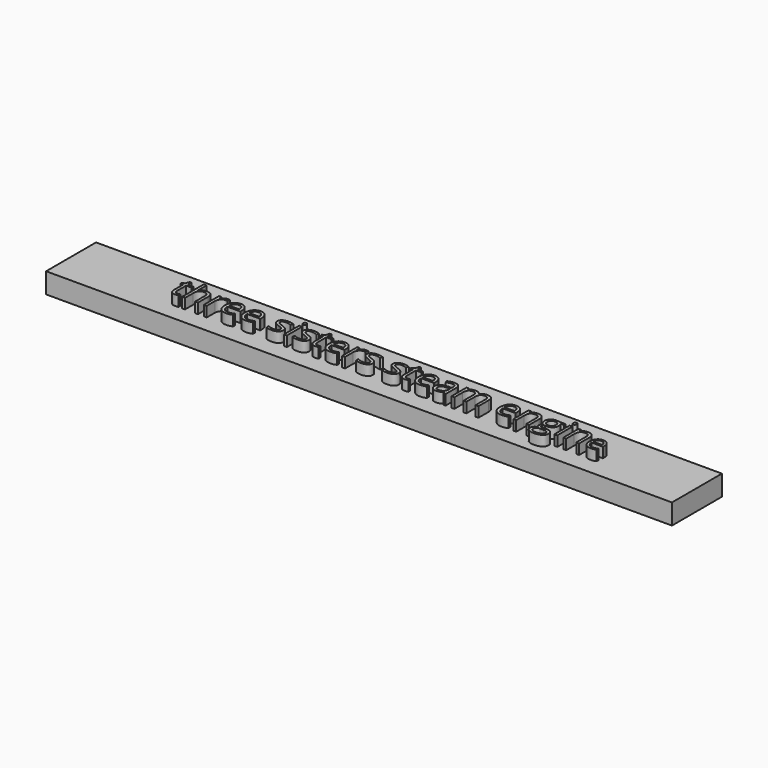
from build123d import *

# Parameters (mm, degrees)
F0_W           = 77.9215320945
F0_H           = 7.7777523547
F0_W_2         = 0.3568928393
F0_H_2         = 2.3552176774
F1_DEPTH       = 2.54
F0_TEXT_SIZE   = 4.4009906964
F0_TEXT_SIZE_2 = 3.8066982395
F2_DEPTH       = 3.81


# Not quite as in the source:
# - Text() gives the source's letters only with a copy of the font that has no kerning and outlines rounded to 1/6400 em; it was checked with that copy


with BuildPart() as f1:
    # F0 (on Top) → F1 (new body)
    with BuildSketch(Plane.XY):
        with Locations((-8.0658122897, -17.1398567036)):
            Rectangle(F0_W, F0_H)
        with BuildLine():
            add(Edge.make_bspline(
                [(-28.4415600998, -16.5940982992), (-28.2565809596, -16.4692889537), (-28.0351561151, -16.4692889537)],
                knots=[0, 0, 0, 1, 1, 1], degree=2))
            add(Edge.make_bspline(
                [(-28.0351561151, -16.4692889537), (-27.8783708216, -16.4692889537), (-27.7539053034, -16.4954198359)],
                knots=[0, 0, 0, 1, 1, 1], degree=2))
            Line((-27.7539053034, -16.4954198359), (-27.8034164488, -16.826181793))
            add(Edge.make_bspline(
                [(-27.8034164488, -16.826181793), (-27.9491992656, -16.7938620175), (-28.0612869974, -16.7938620175)],
                knots=[0, 0, 0, 1, 1, 1], degree=2))
            add(Edge.make_bspline(
                [(-28.0612869974, -16.7938620175), (-28.3473513927, -16.7938620175), (-28.5502095576, -17.0259455113)],
                knots=[0, 0, 0, 1, 1, 1], degree=2))
            add(Edge.make_bspline(
                [(-28.5502095576, -17.0259455113), (-28.7530677225, -17.2580290051), (-28.7530677225, -17.6039193676)],
                knots=[0, 0, 0, 1, 1, 1], degree=2))
            Line((-28.7530677225, -17.6039193676), (-28.7530677225, -18.8678288832))
            Line((-28.7530677225, -18.8678288832), (-29.1099605618, -18.8678288832))
            Line((-29.1099605618, -18.8678288832), (-29.1099605618, -16.5126112059))
            Line((-29.1099605618, -16.5126112059), (-28.815644309, -16.5126112059))
            Line((-28.815644309, -16.5126112059), (-28.7743850212, -16.9485843467))
            Line((-28.7743850212, -16.9485843467), (-28.7571936513, -16.9485843467))
            add(Edge.make_bspline(
                [(-28.7571936513, -16.9485843467), (-28.62653924, -16.7189076447), (-28.4415600998, -16.5940982992)],
                knots=[0, 0, 0, 1, 1, 1], degree=2))
        make_face(mode=Mode.SUBTRACT)
        with BuildLine():
            add(Edge.make_bspline(
                [(-32.8810594648, -18.502340359), (-32.7799742097, -18.6161472278), (-32.6039345819, -18.6161472278)],
                knots=[0, 0, 0, 1, 1, 1], degree=2))
            add(Edge.make_bspline(
                [(-32.6039345819, -18.6161472278), (-32.50903822, -18.6161472278), (-32.421018406, -18.6023941319)],
                knots=[0, 0, 0, 1, 1, 1], degree=2))
            add(Edge.make_bspline(
                [(-32.421018406, -18.6023941319), (-32.3329985921, -18.5886410359), (-32.2814244824, -18.5735126304)],
                knots=[0, 0, 0, 1, 1, 1], degree=2))
            Line((-32.2814244824, -18.5735126304), (-32.2814244824, -18.8465115845))
            add(Edge.make_bspline(
                [(-32.2814244824, -18.8465115845), (-32.3391874853, -18.8740177764), (-32.4519628719, -18.8925844559)],
                knots=[0, 0, 0, 1, 1, 1], degree=2))
            add(Edge.make_bspline(
                [(-32.4519628719, -18.8925844559), (-32.5647382585, -18.9111511354), (-32.6555086916, -18.9111511354)],
                knots=[0, 0, 0, 1, 1, 1], degree=2))
            add(Edge.make_bspline(
                [(-32.6555086916, -18.9111511354), (-33.3383499043, -18.9111511354), (-33.3383499043, -18.1911765637)],
                knots=[0, 0, 0, 1, 1, 1], degree=2))
            Line((-33.3383499043, -18.1911765637), (-33.3383499043, -16.7897360888))
            Line((-33.3383499043, -16.7897360888), (-33.6759884093, -16.7897360888))
            Line((-33.6759884093, -16.7897360888), (-33.6759884093, -16.6178223897))
            Line((-33.6759884093, -16.6178223897), (-33.3383499043, -16.4692889537))
            Line((-33.3383499043, -16.4692889537), (-33.1884411587, -15.9666132976))
            Line((-33.1884411587, -15.9666132976), (-32.9821447198, -15.9666132976))
            Line((-32.9821447198, -15.9666132976), (-32.9821447198, -16.5126112059))
            Line((-32.9821447198, -16.5126112059), (-32.2986158523, -16.5126112059))
            Line((-32.2986158523, -16.5126112059), (-32.2986158523, -16.7897360888))
            Line((-32.2986158523, -16.7897360888), (-32.9821447198, -16.7897360888))
            Line((-32.9821447198, -16.7897360888), (-32.9821447198, -18.1760481581))
            add(Edge.make_bspline(
                [(-32.9821447198, -18.1760481581), (-32.9821447198, -18.3885334902), (-32.8810594648, -18.502340359)],
                knots=[0, 0, 0, 1, 1, 1], degree=2))
        make_face(mode=Mode.SUBTRACT)
        with BuildLine():
            Line((-29.8423129199, -18.8678288832), (-30.1992057591, -18.8678288832))
            Line((-30.1992057591, -18.8678288832), (-30.1992057591, -17.3439858546))
            add(Edge.make_bspline(
                [(-30.1992057591, -17.3439858546), (-30.1992057591, -17.0565461497), (-30.3302039978, -16.9145454343)],
                knots=[0, 0, 0, 1, 1, 1], degree=2))
            add(Edge.make_bspline(
                [(-30.3302039978, -16.9145454343), (-30.4612022365, -16.7725447189), (-30.7410777386, -16.7725447189)],
                knots=[0, 0, 0, 1, 1, 1], degree=2))
            add(Edge.make_bspline(
                [(-30.7410777386, -16.7725447189), (-31.1124113286, -16.7725447189), (-31.2832935455, -16.974715229)],
                knots=[0, 0, 0, 1, 1, 1], degree=2))
            add(Edge.make_bspline(
                [(-31.2832935455, -16.974715229), (-31.4541757624, -17.1768857391), (-31.4541757624, -17.636239143)],
                knots=[0, 0, 0, 1, 1, 1], degree=2))
            Line((-31.4541757624, -17.636239143), (-31.4541757624, -18.8678288832))
            Line((-31.4541757624, -18.8678288832), (-31.8110686017, -18.8678288832))
            Line((-31.8110686017, -18.8678288832), (-31.8110686017, -15.5237636088))
            Line((-31.8110686017, -15.5237636088), (-31.4541757624, -15.5237636088))
            Line((-31.4541757624, -15.5237636088), (-31.4541757624, -16.5359914689))
            add(Edge.make_bspline(
                [(-31.4541757624, -16.5359914689), (-31.4541757624, -16.7189076447), (-31.4713671323, -16.8392472341)],
                knots=[0, 0, 0, 1, 1, 1], degree=2))
            Line((-31.4713671323, -16.8392472341), (-31.4500498336, -16.8392472341))
            add(Edge.make_bspline(
                [(-31.4500498336, -16.8392472341), (-31.3448386498, -16.6693964994), (-31.1502323424, -16.5717495183)],
                knots=[0, 0, 0, 1, 1, 1], degree=2))
            add(Edge.make_bspline(
                [(-31.1502323424, -16.5717495183), (-30.9556260351, -16.4741025373), (-30.7066949988, -16.4741025373)],
                knots=[0, 0, 0, 1, 1, 1], degree=2))
            add(Edge.make_bspline(
                [(-30.7066949988, -16.4741025373), (-30.2748477867, -16.4741025373), (-30.0585803533, -16.679367494)],
                knots=[0, 0, 0, 1, 1, 1], degree=2))
            add(Edge.make_bspline(
                [(-30.0585803533, -16.679367494), (-29.8423129199, -16.8846324507), (-29.8423129199, -17.3316080683)],
                knots=[0, 0, 0, 1, 1, 1], degree=2))
            Line((-29.8423129199, -17.3316080683), (-29.8423129199, -18.8678288832))
        make_face(mode=Mode.SUBTRACT)
        with BuildLine():
            add(Edge.make_bspline(
                [(-25.9109904493, -18.875393086), (-26.0794658744, -18.9111511354), (-26.3180820887, -18.9111511354)],
                knots=[0, 0, 0, 1, 1, 1], degree=2))
            add(Edge.make_bspline(
                [(-26.3180820887, -18.9111511354), (-26.8400120791, -18.9111511354), (-27.1422363621, -18.5927669647)],
                knots=[0, 0, 0, 1, 1, 1], degree=2))
            add(Edge.make_bspline(
                [(-27.1422363621, -18.5927669647), (-27.4444606451, -18.274382794), (-27.4444606451, -17.7098182062)],
                knots=[0, 0, 0, 1, 1, 1], degree=2))
            add(Edge.make_bspline(
                [(-27.4444606451, -17.7098182062), (-27.4444606451, -17.1397523801), (-27.1638974882, -16.8045206669)],
                knots=[0, 0, 0, 1, 1, 1], degree=2))
            add(Edge.make_bspline(
                [(-27.1638974882, -16.8045206669), (-26.8833343313, -16.4692889537), (-26.4102278314, -16.4692889537)],
                knots=[0, 0, 0, 1, 1, 1], degree=2))
            add(Edge.make_bspline(
                [(-26.4102278314, -16.4692889537), (-25.9680657974, -16.4692889537), (-25.7101952488, -16.7605107599)],
                knots=[0, 0, 0, 1, 1, 1], degree=2))
            add(Edge.make_bspline(
                [(-25.7101952488, -16.7605107599), (-25.4523247002, -17.0517325662), (-25.4523247002, -17.5289649948)],
                knots=[0, 0, 0, 1, 1, 1], degree=2))
            Line((-25.4523247002, -17.5289649948), (-25.4523247002, -17.754515768))
            Line((-25.4523247002, -17.754515768), (-27.0745023647, -17.754515768))
            add(Edge.make_bspline(
                [(-27.0745023647, -17.754515768), (-27.0634998879, -18.1691716102), (-26.8647676518, -18.384063734)],
                knots=[0, 0, 0, 1, 1, 1], degree=2))
            add(Edge.make_bspline(
                [(-26.8647676518, -18.384063734), (-26.6660354157, -18.5989558579), (-26.3050166476, -18.5989558579)],
                knots=[0, 0, 0, 1, 1, 1], degree=2))
            add(Edge.make_bspline(
                [(-26.3050166476, -18.5989558579), (-25.9247435452, -18.5989558579), (-25.5534099552, -18.4401075999)],
                knots=[0, 0, 0, 1, 1, 1], degree=2))
            Line((-25.5534099552, -18.4401075999), (-25.5534099552, -18.7584917706))
            add(Edge.make_bspline(
                [(-25.5534099552, -18.7584917706), (-25.7425150242, -18.8396350366), (-25.9109904493, -18.875393086)],
                knots=[0, 0, 0, 1, 1, 1], degree=2))
        make_face(mode=Mode.SUBTRACT)
        with BuildLine():
            add(Edge.make_bspline(
                [(-23.4416220758, -18.875393086), (-23.6100975009, -18.9111511354), (-23.8487137152, -18.9111511354)],
                knots=[0, 0, 0, 1, 1, 1], degree=2))
            add(Edge.make_bspline(
                [(-23.8487137152, -18.9111511354), (-24.3706437056, -18.9111511354), (-24.6728679886, -18.5927669647)],
                knots=[0, 0, 0, 1, 1, 1], degree=2))
            add(Edge.make_bspline(
                [(-24.6728679886, -18.5927669647), (-24.9750922715, -18.274382794), (-24.9750922715, -17.7098182062)],
                knots=[0, 0, 0, 1, 1, 1], degree=2))
            add(Edge.make_bspline(
                [(-24.9750922715, -17.7098182062), (-24.9750922715, -17.1397523801), (-24.6945291146, -16.8045206669)],
                knots=[0, 0, 0, 1, 1, 1], degree=2))
            add(Edge.make_bspline(
                [(-24.6945291146, -16.8045206669), (-24.4139659577, -16.4692889537), (-23.9408594579, -16.4692889537)],
                knots=[0, 0, 0, 1, 1, 1], degree=2))
            add(Edge.make_bspline(
                [(-23.9408594579, -16.4692889537), (-23.4986974238, -16.4692889537), (-23.2408268752, -16.7605107599)],
                knots=[0, 0, 0, 1, 1, 1], degree=2))
            add(Edge.make_bspline(
                [(-23.2408268752, -16.7605107599), (-22.9829563266, -17.0517325662), (-22.9829563266, -17.5289649948)],
                knots=[0, 0, 0, 1, 1, 1], degree=2))
            Line((-22.9829563266, -17.5289649948), (-22.9829563266, -17.754515768))
            Line((-22.9829563266, -17.754515768), (-24.6051339911, -17.754515768))
            add(Edge.make_bspline(
                [(-24.6051339911, -17.754515768), (-24.5941315144, -18.1691716102), (-24.3953992782, -18.384063734)],
                knots=[0, 0, 0, 1, 1, 1], degree=2))
            add(Edge.make_bspline(
                [(-24.3953992782, -18.384063734), (-24.1966670421, -18.5989558579), (-23.835648274, -18.5989558579)],
                knots=[0, 0, 0, 1, 1, 1], degree=2))
            add(Edge.make_bspline(
                [(-23.835648274, -18.5989558579), (-23.4553751717, -18.5989558579), (-23.0840415817, -18.4401075999)],
                knots=[0, 0, 0, 1, 1, 1], degree=2))
            Line((-23.0840415817, -18.4401075999), (-23.0840415817, -18.7584917706))
            add(Edge.make_bspline(
                [(-23.0840415817, -18.7584917706), (-23.2731466507, -18.8396350366), (-23.4416220758, -18.875393086)],
                knots=[0, 0, 0, 1, 1, 1], degree=2))
        make_face(mode=Mode.SUBTRACT)
        with BuildLine():
            add(Edge.make_bspline(
                [(-19.858940587, -17.8363466888), (-19.7117824605, -17.9910690179), (-19.7117824605, -18.2255593035)],
                knots=[0, 0, 0, 1, 1, 1], degree=2))
            add(Edge.make_bspline(
                [(-19.7117824605, -18.2255593035), (-19.7117824605, -18.5542582961), (-19.956587568, -18.7327047158)],
                knots=[0, 0, 0, 1, 1, 1], degree=2))
            add(Edge.make_bspline(
                [(-19.956587568, -18.7327047158), (-20.2013926755, -18.9111511354), (-20.6442423643, -18.9111511354)],
                knots=[0, 0, 0, 1, 1, 1], degree=2))
            add(Edge.make_bspline(
                [(-20.6442423643, -18.9111511354), (-21.1125352806, -18.9111511354), (-21.374531758, -18.7626176994)],
                knots=[0, 0, 0, 1, 1, 1], degree=2))
            Line((-21.374531758, -18.7626176994), (-21.374531758, -18.4318557424))
            add(Edge.make_bspline(
                [(-21.374531758, -18.4318557424), (-21.2046810233, -18.5178125919), (-21.0104185434, -18.5669799098)],
                knots=[0, 0, 0, 1, 1, 1], degree=2))
            add(Edge.make_bspline(
                [(-21.0104185434, -18.5669799098), (-20.8161560634, -18.6161472278), (-20.635302852, -18.6161472278)],
                knots=[0, 0, 0, 1, 1, 1], degree=2))
            add(Edge.make_bspline(
                [(-20.635302852, -18.6161472278), (-20.3561150047, -18.6161472278), (-20.2058624317, -18.5270959317)],
                knots=[0, 0, 0, 1, 1, 1], degree=2))
            add(Edge.make_bspline(
                [(-20.2058624317, -18.5270959317), (-20.0556098587, -18.4380446355), (-20.0556098587, -18.2551284597)],
                knots=[0, 0, 0, 1, 1, 1], degree=2))
            add(Edge.make_bspline(
                [(-20.0556098587, -18.2551284597), (-20.0556098587, -18.1175975005), (-20.1745741385, -18.0199505194)],
                knots=[0, 0, 0, 1, 1, 1], degree=2))
            add(Edge.make_bspline(
                [(-20.1745741385, -18.0199505194), (-20.2935384182, -17.9223035383), (-20.6401164356, -17.7888985078)],
                knots=[0, 0, 0, 1, 1, 1], degree=2))
            add(Edge.make_bspline(
                [(-20.6401164356, -17.7888985078), (-20.9688154282, -17.6664959541), (-21.1073778697, -17.5750378662)],
                knots=[0, 0, 0, 1, 1, 1], degree=2))
            add(Edge.make_bspline(
                [(-21.1073778697, -17.5750378662), (-21.2459403111, -17.4835797782), (-21.3136743086, -17.3677099451)],
                knots=[0, 0, 0, 1, 1, 1], degree=2))
            add(Edge.make_bspline(
                [(-21.3136743086, -17.3677099451), (-21.381408306, -17.2518401119), (-21.381408306, -17.0909288896)],
                knots=[0, 0, 0, 1, 1, 1], degree=2))
            add(Edge.make_bspline(
                [(-21.381408306, -17.0909288896), (-21.381408306, -16.8028015299), (-21.1469180205, -16.6360452418)],
                knots=[0, 0, 0, 1, 1, 1], degree=2))
            add(Edge.make_bspline(
                [(-21.1469180205, -16.6360452418), (-20.9124277349, -16.4692889537), (-20.5046484407, -16.4692889537)],
                knots=[0, 0, 0, 1, 1, 1], degree=2))
            add(Edge.make_bspline(
                [(-20.5046484407, -16.4692889537), (-20.1243753383, -16.4692889537), (-19.7606059511, -16.6240112829)],
                knots=[0, 0, 0, 1, 1, 1], degree=2))
            Line((-19.7606059511, -16.6240112829), (-19.8878220884, -16.9142016069))
            add(Edge.make_bspline(
                [(-19.8878220884, -16.9142016069), (-20.2419643085, -16.7684187901), (-20.5300916682, -16.7684187901)],
                knots=[0, 0, 0, 1, 1, 1], degree=2))
            add(Edge.make_bspline(
                [(-20.5300916682, -16.7684187901), (-20.783836288, -16.7684187901), (-20.9127715623, -16.8478429191)],
                knots=[0, 0, 0, 1, 1, 1], degree=2))
            add(Edge.make_bspline(
                [(-20.9127715623, -16.8478429191), (-21.0417068366, -16.927267048), (-21.0417068366, -17.0668609717)],
                knots=[0, 0, 0, 1, 1, 1], degree=2))
            add(Edge.make_bspline(
                [(-21.0417068366, -17.0668609717), (-21.0417068366, -17.1617573336), (-20.9932271735, -17.2281160214)],
                knots=[0, 0, 0, 1, 1, 1], degree=2))
            add(Edge.make_bspline(
                [(-20.9932271735, -17.2281160214), (-20.9447475103, -17.2944747093), (-20.8374733621, -17.3546445039)],
                knots=[0, 0, 0, 1, 1, 1], degree=2))
            add(Edge.make_bspline(
                [(-20.8374733621, -17.3546445039), (-20.7301992139, -17.4148142986), (-20.4248804843, -17.5289649948)],
                knots=[0, 0, 0, 1, 1, 1], degree=2))
            add(Edge.make_bspline(
                [(-20.4248804843, -17.5289649948), (-20.0060987134, -17.6816243596), (-19.858940587, -17.8363466888)],
                knots=[0, 0, 0, 1, 1, 1], degree=2))
        make_face(mode=Mode.SUBTRACT)
        with Locations((-18.9529553928, -17.6902200445)):
            Rectangle(F0_W_2, F0_H_2, mode=Mode.SUBTRACT)
        with BuildLine():
            add(Edge.make_bspline(
                [(-16.6462173786, -17.8363466888), (-16.4990592522, -17.9910690179), (-16.4990592522, -18.2255593035)],
                knots=[0, 0, 0, 1, 1, 1], degree=2))
            add(Edge.make_bspline(
                [(-16.4990592522, -18.2255593035), (-16.4990592522, -18.5542582961), (-16.7438643596, -18.7327047158)],
                knots=[0, 0, 0, 1, 1, 1], degree=2))
            add(Edge.make_bspline(
                [(-16.7438643596, -18.7327047158), (-16.9886694671, -18.9111511354), (-17.431519156, -18.9111511354)],
                knots=[0, 0, 0, 1, 1, 1], degree=2))
            add(Edge.make_bspline(
                [(-17.431519156, -18.9111511354), (-17.8998120723, -18.9111511354), (-18.1618085496, -18.7626176994)],
                knots=[0, 0, 0, 1, 1, 1], degree=2))
            Line((-18.1618085496, -18.7626176994), (-18.1618085496, -18.4318557424))
            add(Edge.make_bspline(
                [(-18.1618085496, -18.4318557424), (-17.991957815, -18.5178125919), (-17.797695335, -18.5669799098)],
                knots=[0, 0, 0, 1, 1, 1], degree=2))
            add(Edge.make_bspline(
                [(-17.797695335, -18.5669799098), (-17.603432855, -18.6161472278), (-17.4225796436, -18.6161472278)],
                knots=[0, 0, 0, 1, 1, 1], degree=2))
            add(Edge.make_bspline(
                [(-17.4225796436, -18.6161472278), (-17.1433917963, -18.6161472278), (-16.9931392233, -18.5270959317)],
                knots=[0, 0, 0, 1, 1, 1], degree=2))
            add(Edge.make_bspline(
                [(-16.9931392233, -18.5270959317), (-16.8428866503, -18.4380446355), (-16.8428866503, -18.2551284597)],
                knots=[0, 0, 0, 1, 1, 1], degree=2))
            add(Edge.make_bspline(
                [(-16.8428866503, -18.2551284597), (-16.8428866503, -18.1175975005), (-16.9618509301, -18.0199505194)],
                knots=[0, 0, 0, 1, 1, 1], degree=2))
            add(Edge.make_bspline(
                [(-16.9618509301, -18.0199505194), (-17.0808152098, -17.9223035383), (-17.4273932272, -17.7888985078)],
                knots=[0, 0, 0, 1, 1, 1], degree=2))
            add(Edge.make_bspline(
                [(-17.4273932272, -17.7888985078), (-17.7560922198, -17.6664959541), (-17.8946546613, -17.5750378662)],
                knots=[0, 0, 0, 1, 1, 1], degree=2))
            add(Edge.make_bspline(
                [(-17.8946546613, -17.5750378662), (-18.0332171027, -17.4835797782), (-18.1009511002, -17.3677099451)],
                knots=[0, 0, 0, 1, 1, 1], degree=2))
            add(Edge.make_bspline(
                [(-18.1009511002, -17.3677099451), (-18.1686850976, -17.2518401119), (-18.1686850976, -17.0909288896)],
                knots=[0, 0, 0, 1, 1, 1], degree=2))
            add(Edge.make_bspline(
                [(-18.1686850976, -17.0909288896), (-18.1686850976, -16.8028015299), (-17.9341948121, -16.6360452418)],
                knots=[0, 0, 0, 1, 1, 1], degree=2))
            add(Edge.make_bspline(
                [(-17.9341948121, -16.6360452418), (-17.6997045265, -16.4692889537), (-17.2919252323, -16.4692889537)],
                knots=[0, 0, 0, 1, 1, 1], degree=2))
            add(Edge.make_bspline(
                [(-17.2919252323, -16.4692889537), (-16.9116521299, -16.4692889537), (-16.5478827427, -16.6240112829)],
                knots=[0, 0, 0, 1, 1, 1], degree=2))
            Line((-16.5478827427, -16.6240112829), (-16.67509888, -16.9142016069))
            add(Edge.make_bspline(
                [(-16.67509888, -16.9142016069), (-17.0292411001, -16.7684187901), (-17.3173684598, -16.7684187901)],
                knots=[0, 0, 0, 1, 1, 1], degree=2))
            add(Edge.make_bspline(
                [(-17.3173684598, -16.7684187901), (-17.5711130796, -16.7684187901), (-17.7000483539, -16.8478429191)],
                knots=[0, 0, 0, 1, 1, 1], degree=2))
            add(Edge.make_bspline(
                [(-17.7000483539, -16.8478429191), (-17.8289836282, -16.927267048), (-17.8289836282, -17.0668609717)],
                knots=[0, 0, 0, 1, 1, 1], degree=2))
            add(Edge.make_bspline(
                [(-17.8289836282, -17.0668609717), (-17.8289836282, -17.1617573336), (-17.7805039651, -17.2281160214)],
                knots=[0, 0, 0, 1, 1, 1], degree=2))
            add(Edge.make_bspline(
                [(-17.7805039651, -17.2281160214), (-17.7320243019, -17.2944747093), (-17.6247501537, -17.3546445039)],
                knots=[0, 0, 0, 1, 1, 1], degree=2))
            add(Edge.make_bspline(
                [(-17.6247501537, -17.3546445039), (-17.5174760055, -17.4148142986), (-17.2121572759, -17.5289649948)],
                knots=[0, 0, 0, 1, 1, 1], degree=2))
            add(Edge.make_bspline(
                [(-17.2121572759, -17.5289649948), (-16.793375505, -17.6816243596), (-16.6462173786, -17.8363466888)],
                knots=[0, 0, 0, 1, 1, 1], degree=2))
        make_face(mode=Mode.SUBTRACT)
        with BuildLine():
            add(Edge.make_bspline(
                [(-12.9631382895, -18.875393086), (-13.1316137146, -18.9111511354), (-13.3702299289, -18.9111511354)],
                knots=[0, 0, 0, 1, 1, 1], degree=2))
            add(Edge.make_bspline(
                [(-13.3702299289, -18.9111511354), (-13.8921599193, -18.9111511354), (-14.1943842023, -18.5927669647)],
                knots=[0, 0, 0, 1, 1, 1], degree=2))
            add(Edge.make_bspline(
                [(-14.1943842023, -18.5927669647), (-14.4966084853, -18.274382794), (-14.4966084853, -17.7098182062)],
                knots=[0, 0, 0, 1, 1, 1], degree=2))
            add(Edge.make_bspline(
                [(-14.4966084853, -17.7098182062), (-14.4966084853, -17.1397523801), (-14.2160453284, -16.8045206669)],
                knots=[0, 0, 0, 1, 1, 1], degree=2))
            add(Edge.make_bspline(
                [(-14.2160453284, -16.8045206669), (-13.9354821715, -16.4692889537), (-13.4623756716, -16.4692889537)],
                knots=[0, 0, 0, 1, 1, 1], degree=2))
            add(Edge.make_bspline(
                [(-13.4623756716, -16.4692889537), (-13.0202136376, -16.4692889537), (-12.762343089, -16.7605107599)],
                knots=[0, 0, 0, 1, 1, 1], degree=2))
            add(Edge.make_bspline(
                [(-12.762343089, -16.7605107599), (-12.5044725404, -17.0517325662), (-12.5044725404, -17.5289649948)],
                knots=[0, 0, 0, 1, 1, 1], degree=2))
            Line((-12.5044725404, -17.5289649948), (-12.5044725404, -17.754515768))
            Line((-12.5044725404, -17.754515768), (-14.1266502049, -17.754515768))
            add(Edge.make_bspline(
                [(-14.1266502049, -17.754515768), (-14.1156477281, -18.1691716102), (-13.916915492, -18.384063734)],
                knots=[0, 0, 0, 1, 1, 1], degree=2))
            add(Edge.make_bspline(
                [(-13.916915492, -18.384063734), (-13.7181832559, -18.5989558579), (-13.3571644878, -18.5989558579)],
                knots=[0, 0, 0, 1, 1, 1], degree=2))
            add(Edge.make_bspline(
                [(-13.3571644878, -18.5989558579), (-12.9768913854, -18.5989558579), (-12.6055577954, -18.4401075999)],
                knots=[0, 0, 0, 1, 1, 1], degree=2))
            Line((-12.6055577954, -18.4401075999), (-12.6055577954, -18.7584917706))
            add(Edge.make_bspline(
                [(-12.6055577954, -18.7584917706), (-12.7946628644, -18.8396350366), (-12.9631382895, -18.875393086)],
                knots=[0, 0, 0, 1, 1, 1], degree=2))
        make_face(mode=Mode.SUBTRACT)
        with BuildLine():
            add(Edge.make_bspline(
                [(-11.2274975836, -16.5940982992), (-11.0425184434, -16.4692889537), (-10.821093599, -16.4692889537)],
                knots=[0, 0, 0, 1, 1, 1], degree=2))
            add(Edge.make_bspline(
                [(-10.821093599, -16.4692889537), (-10.6643083054, -16.4692889537), (-10.5398427873, -16.4954198359)],
                knots=[0, 0, 0, 1, 1, 1], degree=2))
            Line((-10.5398427873, -16.4954198359), (-10.5893539326, -16.826181793))
            add(Edge.make_bspline(
                [(-10.5893539326, -16.826181793), (-10.7351367494, -16.7938620175), (-10.8472244812, -16.7938620175)],
                knots=[0, 0, 0, 1, 1, 1], degree=2))
            add(Edge.make_bspline(
                [(-10.8472244812, -16.7938620175), (-11.1332888765, -16.7938620175), (-11.3361470414, -17.0259455113)],
                knots=[0, 0, 0, 1, 1, 1], degree=2))
            add(Edge.make_bspline(
                [(-11.3361470414, -17.0259455113), (-11.5390052063, -17.2580290051), (-11.5390052063, -17.6039193676)],
                knots=[0, 0, 0, 1, 1, 1], degree=2))
            Line((-11.5390052063, -17.6039193676), (-11.5390052063, -18.8678288832))
            Line((-11.5390052063, -18.8678288832), (-11.8958980456, -18.8678288832))
            Line((-11.8958980456, -18.8678288832), (-11.8958980456, -16.5126112059))
            Line((-11.8958980456, -16.5126112059), (-11.6015817928, -16.5126112059))
            Line((-11.6015817928, -16.5126112059), (-11.560322505, -16.9485843467))
            Line((-11.560322505, -16.9485843467), (-11.5431311351, -16.9485843467))
            add(Edge.make_bspline(
                [(-11.5431311351, -16.9485843467), (-11.4124767238, -16.7189076447), (-11.2274975836, -16.5940982992)],
                knots=[0, 0, 0, 1, 1, 1], degree=2))
        make_face(mode=Mode.SUBTRACT)
        with BuildLine():
            add(Edge.make_bspline(
                [(-8.7271847442, -17.8363466888), (-8.5800266178, -17.9910690179), (-8.5800266178, -18.2255593035)],
                knots=[0, 0, 0, 1, 1, 1], degree=2))
            add(Edge.make_bspline(
                [(-8.5800266178, -18.2255593035), (-8.5800266178, -18.5542582961), (-8.8248317253, -18.7327047158)],
                knots=[0, 0, 0, 1, 1, 1], degree=2))
            add(Edge.make_bspline(
                [(-8.8248317253, -18.7327047158), (-9.0696368328, -18.9111511354), (-9.5124865216, -18.9111511354)],
                knots=[0, 0, 0, 1, 1, 1], degree=2))
            add(Edge.make_bspline(
                [(-9.5124865216, -18.9111511354), (-9.9807794379, -18.9111511354), (-10.2427759153, -18.7626176994)],
                knots=[0, 0, 0, 1, 1, 1], degree=2))
            Line((-10.2427759153, -18.7626176994), (-10.2427759153, -18.4318557424))
            add(Edge.make_bspline(
                [(-10.2427759153, -18.4318557424), (-10.0729251806, -18.5178125919), (-9.8786627006, -18.5669799098)],
                knots=[0, 0, 0, 1, 1, 1], degree=2))
            add(Edge.make_bspline(
                [(-9.8786627006, -18.5669799098), (-9.6844002207, -18.6161472278), (-9.5035470092, -18.6161472278)],
                knots=[0, 0, 0, 1, 1, 1], degree=2))
            add(Edge.make_bspline(
                [(-9.5035470092, -18.6161472278), (-9.2243591619, -18.6161472278), (-9.0741065889, -18.5270959317)],
                knots=[0, 0, 0, 1, 1, 1], degree=2))
            add(Edge.make_bspline(
                [(-9.0741065889, -18.5270959317), (-8.9238540159, -18.4380446355), (-8.9238540159, -18.2551284597)],
                knots=[0, 0, 0, 1, 1, 1], degree=2))
            add(Edge.make_bspline(
                [(-8.9238540159, -18.2551284597), (-8.9238540159, -18.1175975005), (-9.0428182957, -18.0199505194)],
                knots=[0, 0, 0, 1, 1, 1], degree=2))
            add(Edge.make_bspline(
                [(-9.0428182957, -18.0199505194), (-9.1617825755, -17.9223035383), (-9.5083605928, -17.7888985078)],
                knots=[0, 0, 0, 1, 1, 1], degree=2))
            add(Edge.make_bspline(
                [(-9.5083605928, -17.7888985078), (-9.8370595855, -17.6664959541), (-9.9756220269, -17.5750378662)],
                knots=[0, 0, 0, 1, 1, 1], degree=2))
            add(Edge.make_bspline(
                [(-9.9756220269, -17.5750378662), (-10.1141844684, -17.4835797782), (-10.1819184658, -17.3677099451)],
                knots=[0, 0, 0, 1, 1, 1], degree=2))
            add(Edge.make_bspline(
                [(-10.1819184658, -17.3677099451), (-10.2496524632, -17.2518401119), (-10.2496524632, -17.0909288896)],
                knots=[0, 0, 0, 1, 1, 1], degree=2))
            add(Edge.make_bspline(
                [(-10.2496524632, -17.0909288896), (-10.2496524632, -16.8028015299), (-10.0151621777, -16.6360452418)],
                knots=[0, 0, 0, 1, 1, 1], degree=2))
            add(Edge.make_bspline(
                [(-10.0151621777, -16.6360452418), (-9.7806718922, -16.4692889537), (-9.3728925979, -16.4692889537)],
                knots=[0, 0, 0, 1, 1, 1], degree=2))
            add(Edge.make_bspline(
                [(-9.3728925979, -16.4692889537), (-8.9926194956, -16.4692889537), (-8.6288501083, -16.6240112829)],
                knots=[0, 0, 0, 1, 1, 1], degree=2))
            Line((-8.6288501083, -16.6240112829), (-8.7560662456, -16.9142016069))
            add(Edge.make_bspline(
                [(-8.7560662456, -16.9142016069), (-9.1102084658, -16.7684187901), (-9.3983358254, -16.7684187901)],
                knots=[0, 0, 0, 1, 1, 1], degree=2))
            add(Edge.make_bspline(
                [(-9.3983358254, -16.7684187901), (-9.6520804452, -16.7684187901), (-9.7810157196, -16.8478429191)],
                knots=[0, 0, 0, 1, 1, 1], degree=2))
            add(Edge.make_bspline(
                [(-9.7810157196, -16.8478429191), (-9.9099509939, -16.927267048), (-9.9099509939, -17.0668609717)],
                knots=[0, 0, 0, 1, 1, 1], degree=2))
            add(Edge.make_bspline(
                [(-9.9099509939, -17.0668609717), (-9.9099509939, -17.1617573336), (-9.8614713307, -17.2281160214)],
                knots=[0, 0, 0, 1, 1, 1], degree=2))
            add(Edge.make_bspline(
                [(-9.8614713307, -17.2281160214), (-9.8129916676, -17.2944747093), (-9.7057175194, -17.3546445039)],
                knots=[0, 0, 0, 1, 1, 1], degree=2))
            add(Edge.make_bspline(
                [(-9.7057175194, -17.3546445039), (-9.5984433711, -17.4148142986), (-9.2931246416, -17.5289649948)],
                knots=[0, 0, 0, 1, 1, 1], degree=2))
            add(Edge.make_bspline(
                [(-9.2931246416, -17.5289649948), (-8.8743428706, -17.6816243596), (-8.7271847442, -17.8363466888)],
                knots=[0, 0, 0, 1, 1, 1], degree=2))
        make_face(mode=Mode.SUBTRACT)
        with BuildLine():
            add(Edge.make_bspline(
                [(-15.4352572823, -18.502340359), (-15.3341720272, -18.6161472278), (-15.1581323993, -18.6161472278)],
                knots=[0, 0, 0, 1, 1, 1], degree=2))
            add(Edge.make_bspline(
                [(-15.1581323993, -18.6161472278), (-15.0632360375, -18.6161472278), (-14.9752162235, -18.6023941319)],
                knots=[0, 0, 0, 1, 1, 1], degree=2))
            add(Edge.make_bspline(
                [(-14.9752162235, -18.6023941319), (-14.8871964096, -18.5886410359), (-14.8356222999, -18.5735126304)],
                knots=[0, 0, 0, 1, 1, 1], degree=2))
            Line((-14.8356222999, -18.5735126304), (-14.8356222999, -18.8465115845))
            add(Edge.make_bspline(
                [(-14.8356222999, -18.8465115845), (-14.8933853028, -18.8740177764), (-15.0061606894, -18.8925844559)],
                knots=[0, 0, 0, 1, 1, 1], degree=2))
            add(Edge.make_bspline(
                [(-15.0061606894, -18.8925844559), (-15.118936076, -18.9111511354), (-15.2097065091, -18.9111511354)],
                knots=[0, 0, 0, 1, 1, 1], degree=2))
            add(Edge.make_bspline(
                [(-15.2097065091, -18.9111511354), (-15.8925477218, -18.9111511354), (-15.8925477218, -18.1911765637)],
                knots=[0, 0, 0, 1, 1, 1], degree=2))
            Line((-15.8925477218, -18.1911765637), (-15.8925477218, -16.7897360888))
            Line((-15.8925477218, -16.7897360888), (-16.2301862268, -16.7897360888))
            Line((-16.2301862268, -16.7897360888), (-16.2301862268, -16.6178223897))
            Line((-16.2301862268, -16.6178223897), (-15.8925477218, -16.4692889537))
            Line((-15.8925477218, -16.4692889537), (-15.7426389762, -15.9666132976))
            Line((-15.7426389762, -15.9666132976), (-15.5363425373, -15.9666132976))
            Line((-15.5363425373, -15.9666132976), (-15.5363425373, -16.5126112059))
            Line((-15.5363425373, -16.5126112059), (-14.8528136698, -16.5126112059))
            Line((-14.8528136698, -16.5126112059), (-14.8528136698, -16.7897360888))
            Line((-14.8528136698, -16.7897360888), (-15.5363425373, -16.7897360888))
            Line((-15.5363425373, -16.7897360888), (-15.5363425373, -18.1760481581))
            add(Edge.make_bspline(
                [(-15.5363425373, -18.1760481581), (-15.5363425373, -18.3885334902), (-15.4352572823, -18.502340359)],
                knots=[0, 0, 0, 1, 1, 1], degree=2))
        make_face(mode=Mode.SUBTRACT)
        with BuildLine():
            add(Edge.make_bspline(
                [(-5.4842047248, -17.8363466888), (-5.3370465984, -17.9910690179), (-5.3370465984, -18.2255593035)],
                knots=[0, 0, 0, 1, 1, 1], degree=2))
            add(Edge.make_bspline(
                [(-5.3370465984, -18.2255593035), (-5.3370465984, -18.5542582961), (-5.5818517059, -18.7327047158)],
                knots=[0, 0, 0, 1, 1, 1], degree=2))
            add(Edge.make_bspline(
                [(-5.5818517059, -18.7327047158), (-5.8266568133, -18.9111511354), (-6.2695065022, -18.9111511354)],
                knots=[0, 0, 0, 1, 1, 1], degree=2))
            add(Edge.make_bspline(
                [(-6.2695065022, -18.9111511354), (-6.7377994185, -18.9111511354), (-6.9997958959, -18.7626176994)],
                knots=[0, 0, 0, 1, 1, 1], degree=2))
            Line((-6.9997958959, -18.7626176994), (-6.9997958959, -18.4318557424))
            add(Edge.make_bspline(
                [(-6.9997958959, -18.4318557424), (-6.8299451612, -18.5178125919), (-6.6356826812, -18.5669799098)],
                knots=[0, 0, 0, 1, 1, 1], degree=2))
            add(Edge.make_bspline(
                [(-6.6356826812, -18.5669799098), (-6.4414202013, -18.6161472278), (-6.2605669898, -18.6161472278)],
                knots=[0, 0, 0, 1, 1, 1], degree=2))
            add(Edge.make_bspline(
                [(-6.2605669898, -18.6161472278), (-5.9813791425, -18.6161472278), (-5.8311265695, -18.5270959317)],
                knots=[0, 0, 0, 1, 1, 1], degree=2))
            add(Edge.make_bspline(
                [(-5.8311265695, -18.5270959317), (-5.6808739965, -18.4380446355), (-5.6808739965, -18.2551284597)],
                knots=[0, 0, 0, 1, 1, 1], degree=2))
            add(Edge.make_bspline(
                [(-5.6808739965, -18.2551284597), (-5.6808739965, -18.1175975005), (-5.7998382763, -18.0199505194)],
                knots=[0, 0, 0, 1, 1, 1], degree=2))
            add(Edge.make_bspline(
                [(-5.7998382763, -18.0199505194), (-5.9188025561, -17.9223035383), (-6.2653805734, -17.7888985078)],
                knots=[0, 0, 0, 1, 1, 1], degree=2))
            add(Edge.make_bspline(
                [(-6.2653805734, -17.7888985078), (-6.594079566, -17.6664959541), (-6.7326420075, -17.5750378662)],
                knots=[0, 0, 0, 1, 1, 1], degree=2))
            add(Edge.make_bspline(
                [(-6.7326420075, -17.5750378662), (-6.8712044489, -17.4835797782), (-6.9389384464, -17.3677099451)],
                knots=[0, 0, 0, 1, 1, 1], degree=2))
            add(Edge.make_bspline(
                [(-6.9389384464, -17.3677099451), (-7.0066724438, -17.2518401119), (-7.0066724438, -17.0909288896)],
                knots=[0, 0, 0, 1, 1, 1], degree=2))
            add(Edge.make_bspline(
                [(-7.0066724438, -17.0909288896), (-7.0066724438, -16.8028015299), (-6.7721821583, -16.6360452418)],
                knots=[0, 0, 0, 1, 1, 1], degree=2))
            add(Edge.make_bspline(
                [(-6.7721821583, -16.6360452418), (-6.5376918727, -16.4692889537), (-6.1299125785, -16.4692889537)],
                knots=[0, 0, 0, 1, 1, 1], degree=2))
            add(Edge.make_bspline(
                [(-6.1299125785, -16.4692889537), (-5.7496394762, -16.4692889537), (-5.3858700889, -16.6240112829)],
                knots=[0, 0, 0, 1, 1, 1], degree=2))
            Line((-5.3858700889, -16.6240112829), (-5.5130862262, -16.9142016069))
            add(Edge.make_bspline(
                [(-5.5130862262, -16.9142016069), (-5.8672284463, -16.7684187901), (-6.155355806, -16.7684187901)],
                knots=[0, 0, 0, 1, 1, 1], degree=2))
            add(Edge.make_bspline(
                [(-6.155355806, -16.7684187901), (-6.4091004258, -16.7684187901), (-6.5380357001, -16.8478429191)],
                knots=[0, 0, 0, 1, 1, 1], degree=2))
            add(Edge.make_bspline(
                [(-6.5380357001, -16.8478429191), (-6.6669709744, -16.927267048), (-6.6669709744, -17.0668609717)],
                knots=[0, 0, 0, 1, 1, 1], degree=2))
            add(Edge.make_bspline(
                [(-6.6669709744, -17.0668609717), (-6.6669709744, -17.1617573336), (-6.6184913113, -17.2281160214)],
                knots=[0, 0, 0, 1, 1, 1], degree=2))
            add(Edge.make_bspline(
                [(-6.6184913113, -17.2281160214), (-6.5700116482, -17.2944747093), (-6.4627374999, -17.3546445039)],
                knots=[0, 0, 0, 1, 1, 1], degree=2))
            add(Edge.make_bspline(
                [(-6.4627374999, -17.3546445039), (-6.3554633517, -17.4148142986), (-6.0501446221, -17.5289649948)],
                knots=[0, 0, 0, 1, 1, 1], degree=2))
            add(Edge.make_bspline(
                [(-6.0501446221, -17.5289649948), (-5.6313628512, -17.6816243596), (-5.4842047248, -17.8363466888)],
                knots=[0, 0, 0, 1, 1, 1], degree=2))
        make_face(mode=Mode.SUBTRACT)
        with BuildLine():
            add(Edge.make_bspline(
                [(-1.8011256357, -18.875393086), (-1.9696010608, -18.9111511354), (-2.2082172751, -18.9111511354)],
                knots=[0, 0, 0, 1, 1, 1], degree=2))
            add(Edge.make_bspline(
                [(-2.2082172751, -18.9111511354), (-2.7301472655, -18.9111511354), (-3.0323715485, -18.5927669647)],
                knots=[0, 0, 0, 1, 1, 1], degree=2))
            add(Edge.make_bspline(
                [(-3.0323715485, -18.5927669647), (-3.3345958315, -18.274382794), (-3.3345958315, -17.7098182062)],
                knots=[0, 0, 0, 1, 1, 1], degree=2))
            add(Edge.make_bspline(
                [(-3.3345958315, -17.7098182062), (-3.3345958315, -17.1397523801), (-3.0540326746, -16.8045206669)],
                knots=[0, 0, 0, 1, 1, 1], degree=2))
            add(Edge.make_bspline(
                [(-3.0540326746, -16.8045206669), (-2.7734695177, -16.4692889537), (-2.3003630178, -16.4692889537)],
                knots=[0, 0, 0, 1, 1, 1], degree=2))
            add(Edge.make_bspline(
                [(-2.3003630178, -16.4692889537), (-1.8582009838, -16.4692889537), (-1.6003304352, -16.7605107599)],
                knots=[0, 0, 0, 1, 1, 1], degree=2))
            add(Edge.make_bspline(
                [(-1.6003304352, -16.7605107599), (-1.3424598866, -17.0517325662), (-1.3424598866, -17.5289649948)],
                knots=[0, 0, 0, 1, 1, 1], degree=2))
            Line((-1.3424598866, -17.5289649948), (-1.3424598866, -17.754515768))
            Line((-1.3424598866, -17.754515768), (-2.9646375511, -17.754515768))
            add(Edge.make_bspline(
                [(-2.9646375511, -17.754515768), (-2.9536350743, -18.1691716102), (-2.7549028382, -18.384063734)],
                knots=[0, 0, 0, 1, 1, 1], degree=2))
            add(Edge.make_bspline(
                [(-2.7549028382, -18.384063734), (-2.5561706021, -18.5989558579), (-2.195151834, -18.5989558579)],
                knots=[0, 0, 0, 1, 1, 1], degree=2))
            add(Edge.make_bspline(
                [(-2.195151834, -18.5989558579), (-1.8148787316, -18.5989558579), (-1.4435451416, -18.4401075999)],
                knots=[0, 0, 0, 1, 1, 1], degree=2))
            Line((-1.4435451416, -18.4401075999), (-1.4435451416, -18.7584917706))
            add(Edge.make_bspline(
                [(-1.4435451416, -18.7584917706), (-1.6326502106, -18.8396350366), (-1.8011256357, -18.875393086)],
                knots=[0, 0, 0, 1, 1, 1], degree=2))
        make_face(mode=Mode.SUBTRACT)
        with BuildLine():
            Line((0.9790627058, -18.8678288832), (0.7143156092, -18.8678288832))
            Line((0.7143156092, -18.8678288832), (0.6434871652, -18.5322533426))
            Line((0.6434871652, -18.5322533426), (0.6262957953, -18.5322533426))
            add(Edge.make_bspline(
                [(0.6262957953, -18.5322533426), (0.4502561674, -18.753678187), (0.2752480218, -18.8324146612)],
                knots=[0, 0, 0, 1, 1, 1], degree=2))
            add(Edge.make_bspline(
                [(0.2752480218, -18.8324146612), (0.1002398761, -18.9111511354), (-0.1624442561, -18.9111511354)],
                knots=[0, 0, 0, 1, 1, 1], degree=2))
            add(Edge.make_bspline(
                [(-0.1624442561, -18.9111511354), (-0.5124605474, -18.9111511354), (-0.7111927836, -18.730297924)],
                knots=[0, 0, 0, 1, 1, 1], degree=2))
            add(Edge.make_bspline(
                [(-0.7111927836, -18.730297924), (-0.9099250197, -18.5494447125), (-0.9099250197, -18.2166197911)],
                knots=[0, 0, 0, 1, 1, 1], degree=2))
            add(Edge.make_bspline(
                [(-0.9099250197, -18.2166197911), (-0.9099250197, -17.5035217673), (0.2308942874, -17.4691390275)],
                knots=[0, 0, 0, 1, 1, 1], degree=2))
            Line((0.2308942874, -17.4691390275), (0.6304217241, -17.4560735864))
            Line((0.6304217241, -17.4560735864), (0.6304217241, -17.3096031148))
            add(Edge.make_bspline(
                [(0.6304217241, -17.3096031148), (0.6304217241, -17.0324782319), (0.5114574443, -16.900448511)],
                knots=[0, 0, 0, 1, 1, 1], degree=2))
            add(Edge.make_bspline(
                [(0.5114574443, -16.900448511), (0.3924931645, -16.7684187901), (0.1298090323, -16.7684187901)],
                knots=[0, 0, 0, 1, 1, 1], degree=2))
            add(Edge.make_bspline(
                [(0.1298090323, -16.7684187901), (-0.1645072205, -16.7684187901), (-0.5358408105, -16.9485843467)],
                knots=[0, 0, 0, 1, 1, 1], degree=2))
            Line((-0.5358408105, -16.9485843467), (-0.6458655779, -16.6755853926))
            add(Edge.make_bspline(
                [(-0.6458655779, -16.6755853926), (-0.4718889144, -16.5813766855), (-0.2645609934, -16.5277396114)],
                knots=[0, 0, 0, 1, 1, 1], degree=2))
            add(Edge.make_bspline(
                [(-0.2645609934, -16.5277396114), (-0.0572330723, -16.4741025373), (0.1518139858, -16.4741025373)],
                knots=[0, 0, 0, 1, 1, 1], degree=2))
            add(Edge.make_bspline(
                [(0.1518139858, -16.4741025373), (0.5726587212, -16.4741025373), (0.7758607135, -16.6608008145)],
                knots=[0, 0, 0, 1, 1, 1], degree=2))
            add(Edge.make_bspline(
                [(0.7758607135, -16.6608008145), (0.9790627058, -16.8474990917), (0.9790627058, -17.2600919694)],
                knots=[0, 0, 0, 1, 1, 1], degree=2))
            Line((0.9790627058, -17.2600919694), (0.9790627058, -18.8678288832))
        make_face(mode=Mode.SUBTRACT)
        with BuildLine():
            add(Edge.make_bspline(
                [(-4.2732446285, -18.502340359), (-4.1721593734, -18.6161472278), (-3.9961197456, -18.6161472278)],
                knots=[0, 0, 0, 1, 1, 1], degree=2))
            add(Edge.make_bspline(
                [(-3.9961197456, -18.6161472278), (-3.9012233837, -18.6161472278), (-3.8132035697, -18.6023941319)],
                knots=[0, 0, 0, 1, 1, 1], degree=2))
            add(Edge.make_bspline(
                [(-3.8132035697, -18.6023941319), (-3.7251837558, -18.5886410359), (-3.6736096461, -18.5735126304)],
                knots=[0, 0, 0, 1, 1, 1], degree=2))
            Line((-3.6736096461, -18.5735126304), (-3.6736096461, -18.8465115845))
            add(Edge.make_bspline(
                [(-3.6736096461, -18.8465115845), (-3.731372649, -18.8740177764), (-3.8441480356, -18.8925844559)],
                knots=[0, 0, 0, 1, 1, 1], degree=2))
            add(Edge.make_bspline(
                [(-3.8441480356, -18.8925844559), (-3.9569234222, -18.9111511354), (-4.0476938553, -18.9111511354)],
                knots=[0, 0, 0, 1, 1, 1], degree=2))
            add(Edge.make_bspline(
                [(-4.0476938553, -18.9111511354), (-4.730535068, -18.9111511354), (-4.730535068, -18.1911765637)],
                knots=[0, 0, 0, 1, 1, 1], degree=2))
            Line((-4.730535068, -18.1911765637), (-4.730535068, -16.7897360888))
            Line((-4.730535068, -16.7897360888), (-5.068173573, -16.7897360888))
            Line((-5.068173573, -16.7897360888), (-5.068173573, -16.6178223897))
            Line((-5.068173573, -16.6178223897), (-4.730535068, -16.4692889537))
            Line((-4.730535068, -16.4692889537), (-4.5806263224, -15.9666132976))
            Line((-4.5806263224, -15.9666132976), (-4.3743298835, -15.9666132976))
            Line((-4.3743298835, -15.9666132976), (-4.3743298835, -16.5126112059))
            Line((-4.3743298835, -16.5126112059), (-3.690801016, -16.5126112059))
            Line((-3.690801016, -16.5126112059), (-3.690801016, -16.7897360888))
            Line((-3.690801016, -16.7897360888), (-4.3743298835, -16.7897360888))
            Line((-4.3743298835, -16.7897360888), (-4.3743298835, -18.1760481581))
            add(Edge.make_bspline(
                [(-4.3743298835, -18.1760481581), (-4.3743298835, -18.3885334902), (-4.2732446285, -18.502340359)],
                knots=[0, 0, 0, 1, 1, 1], degree=2))
        make_face(mode=Mode.SUBTRACT)
        with BuildLine():
            Line((5.0719840535, -18.8678288832), (4.715778869, -18.8678288832))
            Line((4.715778869, -18.8678288832), (4.715778869, -17.335733997))
            add(Edge.make_bspline(
                [(4.715778869, -17.335733997), (4.715778869, -17.0537955306), (4.5954392796, -16.9131701247)],
                knots=[0, 0, 0, 1, 1, 1], degree=2))
            add(Edge.make_bspline(
                [(4.5954392796, -16.9131701247), (4.4750996903, -16.7725447189), (4.2213550704, -16.7725447189)],
                knots=[0, 0, 0, 1, 1, 1], degree=2))
            add(Edge.make_bspline(
                [(4.2213550704, -16.7725447189), (3.888530149, -16.7725447189), (3.7293380636, -16.9637127522)],
                knots=[0, 0, 0, 1, 1, 1], degree=2))
            add(Edge.make_bspline(
                [(3.7293380636, -16.9637127522), (3.5701459783, -17.1548807856), (3.5701459783, -17.5523452579)],
                knots=[0, 0, 0, 1, 1, 1], degree=2))
            Line((3.5701459783, -17.5523452579), (3.5701459783, -18.8678288832))
            Line((3.5701459783, -18.8678288832), (3.213253139, -18.8678288832))
            Line((3.213253139, -18.8678288832), (3.213253139, -17.335733997))
            add(Edge.make_bspline(
                [(3.213253139, -17.335733997), (3.213253139, -17.0537955306), (3.0929135497, -16.9131701247)],
                knots=[0, 0, 0, 1, 1, 1], degree=2))
            add(Edge.make_bspline(
                [(3.0929135497, -16.9131701247), (2.9725739603, -16.7725447189), (2.7167663761, -16.7725447189)],
                knots=[0, 0, 0, 1, 1, 1], degree=2))
            add(Edge.make_bspline(
                [(2.7167663761, -16.7725447189), (2.3818784903, -16.7725447189), (2.2261246789, -16.9733399194)],
                knots=[0, 0, 0, 1, 1, 1], degree=2))
            add(Edge.make_bspline(
                [(2.2261246789, -16.9733399194), (2.0703708675, -17.1741351199), (2.0703708675, -17.6321132143)],
                knots=[0, 0, 0, 1, 1, 1], degree=2))
            Line((2.0703708675, -17.6321132143), (2.0703708675, -18.8678288832))
            Line((2.0703708675, -18.8678288832), (1.7134780283, -18.8678288832))
            Line((1.7134780283, -18.8678288832), (1.7134780283, -16.5126112059))
            Line((1.7134780283, -16.5126112059), (2.0036683523, -16.5126112059))
            Line((2.0036683523, -16.5126112059), (2.0614313552, -16.8351213053))
            Line((2.0614313552, -16.8351213053), (2.0786227251, -16.8351213053))
            add(Edge.make_bspline(
                [(2.0786227251, -16.8351213053), (2.1797079802, -16.6632076062), (2.3636556382, -16.56624828)],
                knots=[0, 0, 0, 1, 1, 1], degree=2))
            add(Edge.make_bspline(
                [(2.3636556382, -16.56624828), (2.5476032962, -16.4692889537), (2.7752170338, -16.4692889537)],
                knots=[0, 0, 0, 1, 1, 1], degree=2))
            add(Edge.make_bspline(
                [(2.7752170338, -16.4692889537), (3.3274038352, -16.4692889537), (3.4972545699, -16.8695040451)],
                knots=[0, 0, 0, 1, 1, 1], degree=2))
            Line((3.4972545699, -16.8695040451), (3.5144459398, -16.8695040451))
            add(Edge.make_bspline(
                [(3.5144459398, -16.8695040451), (3.6196571236, -16.6845249049), (3.819420842, -16.5769069293)],
                knots=[0, 0, 0, 1, 1, 1], degree=2))
            add(Edge.make_bspline(
                [(3.819420842, -16.5769069293), (4.0191845603, -16.4692889537), (4.2749921445, -16.4692889537)],
                knots=[0, 0, 0, 1, 1, 1], degree=2))
            add(Edge.make_bspline(
                [(4.2749921445, -16.4692889537), (4.6745195812, -16.4692889537), (4.8732518173, -16.6745539104)],
                knots=[0, 0, 0, 1, 1, 1], degree=2))
            add(Edge.make_bspline(
                [(4.8732518173, -16.6745539104), (5.0719840535, -16.8798188671), (5.0719840535, -17.3316080683)],
                knots=[0, 0, 0, 1, 1, 1], degree=2))
            Line((5.0719840535, -17.3316080683), (5.0719840535, -18.8678288832))
        make_face(mode=Mode.SUBTRACT)
        with BuildLine():
            add(Edge.make_bspline(
                [(8.3527850867, -18.875393086), (8.1843096616, -18.9111511354), (7.9456934473, -18.9111511354)],
                knots=[0, 0, 0, 1, 1, 1], degree=2))
            add(Edge.make_bspline(
                [(7.9456934473, -18.9111511354), (7.4237634569, -18.9111511354), (7.1215391739, -18.5927669647)],
                knots=[0, 0, 0, 1, 1, 1], degree=2))
            add(Edge.make_bspline(
                [(7.1215391739, -18.5927669647), (6.8193148909, -18.274382794), (6.8193148909, -17.7098182062)],
                knots=[0, 0, 0, 1, 1, 1], degree=2))
            add(Edge.make_bspline(
                [(6.8193148909, -17.7098182062), (6.8193148909, -17.1397523801), (7.0998780478, -16.8045206669)],
                knots=[0, 0, 0, 1, 1, 1], degree=2))
            add(Edge.make_bspline(
                [(7.0998780478, -16.8045206669), (7.3804412047, -16.4692889537), (7.8535477045, -16.4692889537)],
                knots=[0, 0, 0, 1, 1, 1], degree=2))
            add(Edge.make_bspline(
                [(7.8535477045, -16.4692889537), (8.2957097386, -16.4692889537), (8.5535802872, -16.7605107599)],
                knots=[0, 0, 0, 1, 1, 1], degree=2))
            add(Edge.make_bspline(
                [(8.5535802872, -16.7605107599), (8.8114508358, -17.0517325662), (8.8114508358, -17.5289649948)],
                knots=[0, 0, 0, 1, 1, 1], degree=2))
            Line((8.8114508358, -17.5289649948), (8.8114508358, -17.754515768))
            Line((8.8114508358, -17.754515768), (7.1892731713, -17.754515768))
            add(Edge.make_bspline(
                [(7.1892731713, -17.754515768), (7.200275648, -18.1691716102), (7.3990078842, -18.384063734)],
                knots=[0, 0, 0, 1, 1, 1], degree=2))
            add(Edge.make_bspline(
                [(7.3990078842, -18.384063734), (7.5977401203, -18.5989558579), (7.9587588884, -18.5989558579)],
                knots=[0, 0, 0, 1, 1, 1], degree=2))
            add(Edge.make_bspline(
                [(7.9587588884, -18.5989558579), (8.3390319907, -18.5989558579), (8.7103655808, -18.4401075999)],
                knots=[0, 0, 0, 1, 1, 1], degree=2))
            Line((8.7103655808, -18.4401075999), (8.7103655808, -18.7584917706))
            add(Edge.make_bspline(
                [(8.7103655808, -18.7584917706), (8.5212605118, -18.8396350366), (8.3527850867, -18.875393086)],
                knots=[0, 0, 0, 1, 1, 1], degree=2))
        make_face(mode=Mode.SUBTRACT)
        with BuildLine():
            Line((11.3887810124, -18.8678288832), (11.0318881731, -18.8678288832))
            Line((11.0318881731, -18.8678288832), (11.0318881731, -17.3439858546))
            add(Edge.make_bspline(
                [(11.0318881731, -17.3439858546), (11.0318881731, -17.0565461497), (10.9008899344, -16.9145454343)],
                knots=[0, 0, 0, 1, 1, 1], degree=2))
            add(Edge.make_bspline(
                [(10.9008899344, -16.9145454343), (10.7698916957, -16.7725447189), (10.4900161936, -16.7725447189)],
                knots=[0, 0, 0, 1, 1, 1], degree=2))
            add(Edge.make_bspline(
                [(10.4900161936, -16.7725447189), (10.120745568, -16.7725447189), (9.9488318689, -16.9723084372)],
                knots=[0, 0, 0, 1, 1, 1], degree=2))
            add(Edge.make_bspline(
                [(9.9488318689, -16.9723084372), (9.7769181698, -17.1720721555), (9.7769181698, -17.6321132143)],
                knots=[0, 0, 0, 1, 1, 1], degree=2))
            Line((9.7769181698, -17.6321132143), (9.7769181698, -18.8678288832))
            Line((9.7769181698, -18.8678288832), (9.4200253306, -18.8678288832))
            Line((9.4200253306, -18.8678288832), (9.4200253306, -16.5126112059))
            Line((9.4200253306, -16.5126112059), (9.7102156546, -16.5126112059))
            Line((9.7102156546, -16.5126112059), (9.7679786575, -16.8351213053))
            Line((9.7679786575, -16.8351213053), (9.7851700274, -16.8351213053))
            add(Edge.make_bspline(
                [(9.7851700274, -16.8351213053), (9.8951947948, -16.6611446419), (10.0928955487, -16.5652167978)],
                knots=[0, 0, 0, 1, 1, 1], degree=2))
            add(Edge.make_bspline(
                [(10.0928955487, -16.5652167978), (10.2905963027, -16.4692889537), (10.5333384458, -16.4692889537)],
                knots=[0, 0, 0, 1, 1, 1], degree=2))
            add(Edge.make_bspline(
                [(10.5333384458, -16.4692889537), (10.9589967647, -16.4692889537), (11.1738888886, -16.6745539104)],
                knots=[0, 0, 0, 1, 1, 1], degree=2))
            add(Edge.make_bspline(
                [(11.1738888886, -16.6745539104), (11.3887810124, -16.8798188671), (11.3887810124, -17.3316080683)],
                knots=[0, 0, 0, 1, 1, 1], degree=2))
            Line((11.3887810124, -17.3316080683), (11.3887810124, -18.8678288832))
        make_face(mode=Mode.SUBTRACT)
        with BuildLine():
            Line((13.2344464857, -16.5126112059), (14.0486297646, -16.5126112059))
            Line((14.0486297646, -16.5126112059), (14.0486297646, -16.738161979))
            Line((14.0486297646, -16.738161979), (13.6126566237, -16.7897360888))
            add(Edge.make_bspline(
                [(13.6126566237, -16.7897360888), (13.672482591, -16.8646904616), (13.7199307719, -16.9864053605)],
                knots=[0, 0, 0, 1, 1, 1], degree=2))
            add(Edge.make_bspline(
                [(13.7199307719, -16.9864053605), (13.7673789529, -17.1081202595), (13.7673789529, -17.2600919694)],
                knots=[0, 0, 0, 1, 1, 1], degree=2))
            add(Edge.make_bspline(
                [(13.7673789529, -17.2600919694), (13.7673789529, -17.6066699868), (13.5308257029, -17.8129664257)],
                knots=[0, 0, 0, 1, 1, 1], degree=2))
            add(Edge.make_bspline(
                [(13.5308257029, -17.8129664257), (13.294272453, -18.0192628646), (12.8816795752, -18.0192628646)],
                knots=[0, 0, 0, 1, 1, 1], degree=2))
            add(Edge.make_bspline(
                [(12.8816795752, -18.0192628646), (12.7764683914, -18.0192628646), (12.6843226487, -18.0020714947)],
                knots=[0, 0, 0, 1, 1, 1], degree=2))
            add(Edge.make_bspline(
                [(12.6843226487, -18.0020714947), (12.4567089111, -18.122411084), (12.4567089111, -18.304639605)],
                knots=[0, 0, 0, 1, 1, 1], degree=2))
            add(Edge.make_bspline(
                [(12.4567089111, -18.304639605), (12.4567089111, -18.4015989313), (12.5361330401, -18.4476718027)],
                knots=[0, 0, 0, 1, 1, 1], degree=2))
            add(Edge.make_bspline(
                [(12.5361330401, -18.4476718027), (12.615557169, -18.493744674), (12.8087881668, -18.493744674)],
                knots=[0, 0, 0, 1, 1, 1], degree=2))
            Line((12.8087881668, -18.493744674), (13.2255069734, -18.493744674))
            add(Edge.make_bspline(
                [(13.2255069734, -18.493744674), (13.6085306949, -18.493744674), (13.8134518242, -18.6549997238)],
                knots=[0, 0, 0, 1, 1, 1], degree=2))
            add(Edge.make_bspline(
                [(13.8134518242, -18.6549997238), (14.0183729535, -18.8162547735), (14.0183729535, -19.1236364675)],
                knots=[0, 0, 0, 1, 1, 1], degree=2))
            add(Edge.make_bspline(
                [(14.0183729535, -19.1236364675), (14.0183729535, -19.5149120466), (13.7048023664, -19.7201770033)],
                knots=[0, 0, 0, 1, 1, 1], degree=2))
            add(Edge.make_bspline(
                [(13.7048023664, -19.7201770033), (13.3912317793, -19.92544196), (12.7895338325, -19.92544196)],
                knots=[0, 0, 0, 1, 1, 1], degree=2))
            add(Edge.make_bspline(
                [(12.7895338325, -19.92544196), (12.3274298094, -19.92544196), (12.0771234635, -19.7535282609)],
                knots=[0, 0, 0, 1, 1, 1], degree=2))
            add(Edge.make_bspline(
                [(12.0771234635, -19.7535282609), (11.8268171177, -19.5816145618), (11.8268171177, -19.2673563199)],
                knots=[0, 0, 0, 1, 1, 1], degree=2))
            add(Edge.make_bspline(
                [(11.8268171177, -19.2673563199), (11.8268171177, -19.0528080234), (11.9643480769, -18.8956789025)],
                knots=[0, 0, 0, 1, 1, 1], degree=2))
            add(Edge.make_bspline(
                [(11.9643480769, -18.8956789025), (12.1018790362, -18.7385497815), (12.3508100724, -18.682849743)],
                knots=[0, 0, 0, 1, 1, 1], degree=2))
            add(Edge.make_bspline(
                [(12.3508100724, -18.682849743), (12.2607272941, -18.64227811), (12.1995260173, -18.5563212605)],
                knots=[0, 0, 0, 1, 1, 1], degree=2))
            add(Edge.make_bspline(
                [(12.1995260173, -18.5563212605), (12.1383247404, -18.470364411), (12.1383247404, -18.3562137148)],
                knots=[0, 0, 0, 1, 1, 1], degree=2))
            add(Edge.make_bspline(
                [(12.1383247404, -18.3562137148), (12.1383247404, -18.2276222679), (12.20709022, -18.1306629416)],
                knots=[0, 0, 0, 1, 1, 1], degree=2))
            add(Edge.make_bspline(
                [(12.20709022, -18.1306629416), (12.2758556997, -18.0337036153), (12.4243891357, -17.943620837)],
                knots=[0, 0, 0, 1, 1, 1], degree=2))
            add(Edge.make_bspline(
                [(12.4243891357, -17.943620837), (12.2414729598, -17.8686664642), (12.1266346089, -17.6881570802)],
                knots=[0, 0, 0, 1, 1, 1], degree=2))
            add(Edge.make_bspline(
                [(12.1266346089, -17.6881570802), (12.0117962579, -17.5076476961), (12.0117962579, -17.275220375)],
                knots=[0, 0, 0, 1, 1, 1], degree=2))
            add(Edge.make_bspline(
                [(12.0117962579, -17.275220375), (12.0117962579, -16.8887583794), (12.2438797516, -16.6790236666)],
                knots=[0, 0, 0, 1, 1, 1], degree=2))
            add(Edge.make_bspline(
                [(12.2438797516, -16.6790236666), (12.4759632454, -16.4692889537), (12.9009339095, -16.4692889537)],
                knots=[0, 0, 0, 1, 1, 1], degree=2))
            add(Edge.make_bspline(
                [(12.9009339095, -16.4692889537), (13.0859130497, -16.4692889537), (13.2344464857, -16.5126112059)],
                knots=[0, 0, 0, 1, 1, 1], degree=2))
        make_face(mode=Mode.SUBTRACT)
        with Locations((14.710497506, -17.6902200445)):
            Rectangle(F0_W_2, F0_H_2, mode=Mode.SUBTRACT)
        with BuildLine():
            add(Edge.make_bspline(
                [(19.4572746065, -18.9397588725), (19.3115494395, -18.9706882957), (19.1051550193, -18.9706882957)],
                knots=[0, 0, 0, 1, 1, 1], degree=2))
            add(Edge.make_bspline(
                [(19.1051550193, -18.9706882957), (18.6537044, -18.9706882957), (18.3922912943, -18.6952974699)],
                knots=[0, 0, 0, 1, 1, 1], degree=2))
            add(Edge.make_bspline(
                [(18.3922912943, -18.6952974699), (18.1308781887, -18.4199066441), (18.1308781887, -17.9315786356)],
                knots=[0, 0, 0, 1, 1, 1], degree=2))
            add(Edge.make_bspline(
                [(18.1308781887, -17.9315786356), (18.1308781887, -17.4384922543), (18.3735552014, -17.1485289118)],
                knots=[0, 0, 0, 1, 1, 1], degree=2))
            add(Edge.make_bspline(
                [(18.3735552014, -17.1485289118), (18.6162322142, -16.8585655693), (19.0254522749, -16.8585655693)],
                knots=[0, 0, 0, 1, 1, 1], degree=2))
            add(Edge.make_bspline(
                [(19.0254522749, -16.8585655693), (19.4079064887, -16.8585655693), (19.6309552137, -17.1104619294)],
                knots=[0, 0, 0, 1, 1, 1], degree=2))
            add(Edge.make_bspline(
                [(19.6309552137, -17.1104619294), (19.8540039386, -17.3623582895), (19.8540039386, -17.7751471298)],
                knots=[0, 0, 0, 1, 1, 1], degree=2))
            Line((19.8540039386, -17.7751471298), (19.8540039386, -17.9702404146))
            Line((19.8540039386, -17.9702404146), (18.4508787594, -17.9702404146))
            add(Edge.make_bspline(
                [(18.4508787594, -17.9702404146), (18.460395505, -18.3289027643), (18.6322917224, -18.5147767018)],
                knots=[0, 0, 0, 1, 1, 1], degree=2))
            add(Edge.make_bspline(
                [(18.6322917224, -18.5147767018), (18.8041879398, -18.7006506393), (19.1164561547, -18.7006506393)],
                knots=[0, 0, 0, 1, 1, 1], degree=2))
            add(Edge.make_bspline(
                [(19.1164561547, -18.7006506393), (19.4453786745, -18.7006506393), (19.7665688385, -18.5632526247)],
                knots=[0, 0, 0, 1, 1, 1], degree=2))
            Line((19.7665688385, -18.5632526247), (19.7665688385, -18.8386434505))
            add(Edge.make_bspline(
                [(19.7665688385, -18.8386434505), (19.6029997735, -18.9088294493), (19.4572746065, -18.9397588725)],
                knots=[0, 0, 0, 1, 1, 1], degree=2))
        make_face(mode=Mode.SUBTRACT)
        with BuildLine():
            Line((17.6141198834, -18.8678288832), (17.2572270442, -18.8678288832))
            Line((17.2572270442, -18.8678288832), (17.2572270442, -17.3439858546))
            add(Edge.make_bspline(
                [(17.2572270442, -17.3439858546), (17.2572270442, -17.0565461497), (17.1262288055, -16.9145454343)],
                knots=[0, 0, 0, 1, 1, 1], degree=2))
            add(Edge.make_bspline(
                [(17.1262288055, -16.9145454343), (16.9952305668, -16.7725447189), (16.7153550647, -16.7725447189)],
                knots=[0, 0, 0, 1, 1, 1], degree=2))
            add(Edge.make_bspline(
                [(16.7153550647, -16.7725447189), (16.346084439, -16.7725447189), (16.17417074, -16.9723084372)],
                knots=[0, 0, 0, 1, 1, 1], degree=2))
            add(Edge.make_bspline(
                [(16.17417074, -16.9723084372), (16.0022570409, -17.1720721555), (16.0022570409, -17.6321132143)],
                knots=[0, 0, 0, 1, 1, 1], degree=2))
            Line((16.0022570409, -17.6321132143), (16.0022570409, -18.8678288832))
            Line((16.0022570409, -18.8678288832), (15.6453642016, -18.8678288832))
            Line((15.6453642016, -18.8678288832), (15.6453642016, -16.5126112059))
            Line((15.6453642016, -16.5126112059), (15.9355545256, -16.5126112059))
            Line((15.9355545256, -16.5126112059), (15.9933175285, -16.8351213053))
            Line((15.9933175285, -16.8351213053), (16.0105088984, -16.8351213053))
            add(Edge.make_bspline(
                [(16.0105088984, -16.8351213053), (16.1205336658, -16.6611446419), (16.3182344198, -16.5652167978)],
                knots=[0, 0, 0, 1, 1, 1], degree=2))
            add(Edge.make_bspline(
                [(16.3182344198, -16.5652167978), (16.5159351737, -16.4692889537), (16.7586773168, -16.4692889537)],
                knots=[0, 0, 0, 1, 1, 1], degree=2))
            add(Edge.make_bspline(
                [(16.7586773168, -16.4692889537), (17.1843356357, -16.4692889537), (17.3992277596, -16.6745539104)],
                knots=[0, 0, 0, 1, 1, 1], degree=2))
            add(Edge.make_bspline(
                [(17.3992277596, -16.6745539104), (17.6141198834, -16.8798188671), (17.6141198834, -17.3316080683)],
                knots=[0, 0, 0, 1, 1, 1], degree=2))
            Line((17.6141198834, -17.3316080683), (17.6141198834, -18.8678288832))
        make_face(mode=Mode.SUBTRACT)
        with BuildLine():
            add(Edge.make_bspline(
                [(-19.1014888288, -16.0539454567), (-19.1616586235, -15.9948071442), (-19.1616586235, -15.8744675549)],
                knots=[0, 0, 0, 1, 1, 1], degree=2))
            add(Edge.make_bspline(
                [(-19.1616586235, -15.8744675549), (-19.1616586235, -15.7520650011), (-19.1014888288, -15.694989653)],
                knots=[0, 0, 0, 1, 1, 1], degree=2))
            add(Edge.make_bspline(
                [(-19.1014888288, -15.694989653), (-19.0413190341, -15.6379143049), (-18.950548601, -15.6379143049)],
                knots=[0, 0, 0, 1, 1, 1], degree=2))
            add(Edge.make_bspline(
                [(-18.950548601, -15.6379143049), (-18.8645917515, -15.6379143049), (-18.8023589924, -15.6960211352)],
                knots=[0, 0, 0, 1, 1, 1], degree=2))
            add(Edge.make_bspline(
                [(-18.8023589924, -15.6960211352), (-18.7401262333, -15.7541279655), (-18.7401262333, -15.8744675549)],
                knots=[0, 0, 0, 1, 1, 1], degree=2))
            add(Edge.make_bspline(
                [(-18.7401262333, -15.8744675549), (-18.7401262333, -15.9948071442), (-18.8023589924, -16.0539454567)],
                knots=[0, 0, 0, 1, 1, 1], degree=2))
            add(Edge.make_bspline(
                [(-18.8023589924, -16.0539454567), (-18.8645917515, -16.1130837692), (-18.950548601, -16.1130837692)],
                knots=[0, 0, 0, 1, 1, 1], degree=2))
            add(Edge.make_bspline(
                [(-18.950548601, -16.1130837692), (-19.0413190341, -16.1130837692), (-19.1014888288, -16.0539454567)],
                knots=[0, 0, 0, 1, 1, 1], degree=2))
        make_face(mode=Mode.SUBTRACT)
        with BuildLine():
            add(Edge.make_bspline(
                [(14.56196407, -16.0539454567), (14.5017942753, -15.9948071442), (14.5017942753, -15.8744675549)],
                knots=[0, 0, 0, 1, 1, 1], degree=2))
            add(Edge.make_bspline(
                [(14.5017942753, -15.8744675549), (14.5017942753, -15.7520650011), (14.56196407, -15.694989653)],
                knots=[0, 0, 0, 1, 1, 1], degree=2))
            add(Edge.make_bspline(
                [(14.56196407, -15.694989653), (14.6221338647, -15.6379143049), (14.7129042978, -15.6379143049)],
                knots=[0, 0, 0, 1, 1, 1], degree=2))
            add(Edge.make_bspline(
                [(14.7129042978, -15.6379143049), (14.7988611473, -15.6379143049), (14.8610939064, -15.6960211352)],
                knots=[0, 0, 0, 1, 1, 1], degree=2))
            add(Edge.make_bspline(
                [(14.8610939064, -15.6960211352), (14.9233266655, -15.7541279655), (14.9233266655, -15.8744675549)],
                knots=[0, 0, 0, 1, 1, 1], degree=2))
            add(Edge.make_bspline(
                [(14.9233266655, -15.8744675549), (14.9233266655, -15.9948071442), (14.8610939064, -16.0539454567)],
                knots=[0, 0, 0, 1, 1, 1], degree=2))
            add(Edge.make_bspline(
                [(14.8610939064, -16.0539454567), (14.7988611473, -16.1130837692), (14.7129042978, -16.1130837692)],
                knots=[0, 0, 0, 1, 1, 1], degree=2))
            add(Edge.make_bspline(
                [(14.7129042978, -16.1130837692), (14.6221338647, -16.1130837692), (14.56196407, -16.0539454567)],
                knots=[0, 0, 0, 1, 1, 1], degree=2))
        make_face(mode=Mode.SUBTRACT)
    extrude(amount=F1_DEPTH)


with BuildPart() as f1b:
    # F0 (on Top) → F1, piece 2 (new body)
    with BuildSketch(Plane.XY):
        with BuildLine():
            add(Edge.make_bspline(
                [(-0.4189394951, -18.5154058001), (-0.3020381797, -18.6161472278), (-0.0916158121, -18.6161472278)],
                knots=[0, 0, 0, 1, 1, 1], degree=2))
            add(Edge.make_bspline(
                [(-0.0916158121, -18.6161472278), (0.2418967641, -18.6161472278), (0.4320333153, -18.4335748794)],
                knots=[0, 0, 0, 1, 1, 1], degree=2))
            add(Edge.make_bspline(
                [(0.4320333153, -18.4335748794), (0.6221698665, -18.2510025309), (0.6221698665, -17.9223035383)],
                knots=[0, 0, 0, 1, 1, 1], degree=2))
            Line((0.6221698665, -17.9223035383), (0.6221698665, -17.7098182062))
            Line((0.6221698665, -17.7098182062), (0.2652770272, -17.724258957))
            add(Edge.make_bspline(
                [(0.2652770272, -17.724258957), (-0.1603812917, -17.7393873625), (-0.3481110511, -17.8566325052)],
                knots=[0, 0, 0, 1, 1, 1], degree=2))
            add(Edge.make_bspline(
                [(-0.3481110511, -17.8566325052), (-0.5358408105, -17.973877648), (-0.5358408105, -18.2207457199)],
                knots=[0, 0, 0, 1, 1, 1], degree=2))
            add(Edge.make_bspline(
                [(-0.5358408105, -18.2207457199), (-0.5358408105, -18.4146643725), (-0.4189394951, -18.5154058001)],
                knots=[0, 0, 0, 1, 1, 1], degree=2))
        make_face()
    extrude(amount=F1_DEPTH)


with BuildPart() as f1c:
    # F0 (on Top) → F1, piece 3 (new body)
    with BuildSketch(Plane.XY):
        with BuildLine():
            add(Edge.make_bspline(
                [(-13.0370611801, -16.9478966919), (-13.1873137531, -16.7684187901), (-13.4671892552, -16.7684187901)],
                knots=[0, 0, 0, 1, 1, 1], degree=2))
            add(Edge.make_bspline(
                [(-13.4671892552, -16.7684187901), (-13.7505030313, -16.7684187901), (-13.9193222838, -16.9530541029)],
                knots=[0, 0, 0, 1, 1, 1], degree=2))
            add(Edge.make_bspline(
                [(-13.9193222838, -16.9530541029), (-14.0881415363, -17.1376894157), (-14.1183983473, -17.464325444)],
                knots=[0, 0, 0, 1, 1, 1], degree=2))
            Line((-14.1183983473, -17.464325444), (-12.8868086071, -17.464325444))
            add(Edge.make_bspline(
                [(-12.8868086071, -17.464325444), (-12.8868086071, -17.1273745938), (-13.0370611801, -16.9478966919)],
                knots=[0, 0, 0, 1, 1, 1], degree=2))
        make_face()
    extrude(amount=F1_DEPTH)


with BuildPart() as f1d:
    # F0 (on Top) → F1, piece 4 (new body)
    with BuildSketch(Plane.XY):
        with BuildLine():
            add(Edge.make_bspline(
                [(-23.5155449664, -16.9478966919), (-23.6657975394, -16.7684187901), (-23.9456730415, -16.7684187901)],
                knots=[0, 0, 0, 1, 1, 1], degree=2))
            add(Edge.make_bspline(
                [(-23.9456730415, -16.7684187901), (-24.2289868175, -16.7684187901), (-24.39780607, -16.9530541029)],
                knots=[0, 0, 0, 1, 1, 1], degree=2))
            add(Edge.make_bspline(
                [(-24.39780607, -16.9530541029), (-24.5666253225, -17.1376894157), (-24.5968821336, -17.464325444)],
                knots=[0, 0, 0, 1, 1, 1], degree=2))
            Line((-24.5968821336, -17.464325444), (-23.3652923934, -17.464325444))
            add(Edge.make_bspline(
                [(-23.3652923934, -17.464325444), (-23.3652923934, -17.1273745938), (-23.5155449664, -16.9478966919)],
                knots=[0, 0, 0, 1, 1, 1], degree=2))
        make_face()
    extrude(amount=F1_DEPTH)


with BuildPart() as f1e:
    # F0 (on Top) → F1, piece 5 (new body)
    with BuildSketch(Plane.XY):
        with BuildLine():
            add(Edge.make_bspline(
                [(-25.9849133399, -16.9478966919), (-26.1351659129, -16.7684187901), (-26.415041415, -16.7684187901)],
                knots=[0, 0, 0, 1, 1, 1], degree=2))
            add(Edge.make_bspline(
                [(-26.415041415, -16.7684187901), (-26.6983551911, -16.7684187901), (-26.8671744436, -16.9530541029)],
                knots=[0, 0, 0, 1, 1, 1], degree=2))
            add(Edge.make_bspline(
                [(-26.8671744436, -16.9530541029), (-27.0359936961, -17.1376894157), (-27.0662505071, -17.464325444)],
                knots=[0, 0, 0, 1, 1, 1], degree=2))
            Line((-27.0662505071, -17.464325444), (-25.8346607669, -17.464325444))
            add(Edge.make_bspline(
                [(-25.8346607669, -17.464325444), (-25.8346607669, -17.1273745938), (-25.9849133399, -16.9478966919)],
                knots=[0, 0, 0, 1, 1, 1], degree=2))
        make_face()
    extrude(amount=F1_DEPTH)


with BuildPart() as f1f:
    # F0 (on Top) → F1, piece 6 (new body)
    with BuildSketch(Plane.XY):
        with BuildLine():
            add(Edge.make_bspline(
                [(12.4993435085, -16.865034289), (12.3638755136, -17.0001584564), (12.3638755136, -17.2669685174)],
                knots=[0, 0, 0, 1, 1, 1], degree=2))
            add(Edge.make_bspline(
                [(12.3638755136, -17.2669685174), (12.3638755136, -17.5138365893), (12.5034694372, -17.6407088992)],
                knots=[0, 0, 0, 1, 1, 1], degree=2))
            add(Edge.make_bspline(
                [(12.5034694372, -17.6407088992), (12.6430633609, -17.7675812091), (12.8926820519, -17.7675812091)],
                knots=[0, 0, 0, 1, 1, 1], degree=2))
            add(Edge.make_bspline(
                [(12.8926820519, -17.7675812091), (13.4146120423, -17.7675812091), (13.4146120423, -17.2600919694)],
                knots=[0, 0, 0, 1, 1, 1], degree=2))
            add(Edge.make_bspline(
                [(13.4146120423, -17.2600919694), (13.4146120423, -16.7299101215), (12.8864931588, -16.7299101215)],
                knots=[0, 0, 0, 1, 1, 1], degree=2))
            add(Edge.make_bspline(
                [(12.8864931588, -16.7299101215), (12.6348115033, -16.7299101215), (12.4993435085, -16.865034289)],
                knots=[0, 0, 0, 1, 1, 1], degree=2))
        make_face()
    extrude(amount=F1_DEPTH)


with BuildPart() as f1g:
    # F0 (on Top) → F1, piece 7 (new body)
    with BuildSketch(Plane.XY):
        with BuildLine():
            add(Edge.make_bspline(
                [(12.3061125107, -18.9300616423), (12.1706445158, -19.0459314755), (12.1706445158, -19.2632303911)],
                knots=[0, 0, 0, 1, 1, 1], degree=2))
            add(Edge.make_bspline(
                [(12.1706445158, -19.2632303911), (12.1706445158, -19.4543984245), (12.3318995656, -19.5534207152)],
                knots=[0, 0, 0, 1, 1, 1], degree=2))
            add(Edge.make_bspline(
                [(12.3318995656, -19.5534207152), (12.4931546153, -19.6524430058), (12.7936597613, -19.6524430058)],
                knots=[0, 0, 0, 1, 1, 1], degree=2))
            add(Edge.make_bspline(
                [(12.7936597613, -19.6524430058), (13.2426983433, -19.6524430058), (13.4586219493, -19.5180064931)],
                knots=[0, 0, 0, 1, 1, 1], degree=2))
            add(Edge.make_bspline(
                [(13.4586219493, -19.5180064931), (13.6745455554, -19.3835699805), (13.6745455554, -19.1538932785)],
                knots=[0, 0, 0, 1, 1, 1], degree=2))
            add(Edge.make_bspline(
                [(13.6745455554, -19.1538932785), (13.6745455554, -18.9627252451), (13.5566127578, -18.8884585271)],
                knots=[0, 0, 0, 1, 1, 1], degree=2))
            add(Edge.make_bspline(
                [(13.5566127578, -18.8884585271), (13.4386799602, -18.8141918091), (13.112043932, -18.8141918091)],
                knots=[0, 0, 0, 1, 1, 1], degree=2))
            Line((13.112043932, -18.8141918091), (12.6843226487, -18.8141918091))
            add(Edge.make_bspline(
                [(12.6843226487, -18.8141918091), (12.4415805056, -18.8141918091), (12.3061125107, -18.9300616423)],
                knots=[0, 0, 0, 1, 1, 1], degree=2))
        make_face()
    extrude(amount=F1_DEPTH)


with BuildPart() as f1h:
    # F0 (on Top) → F1, piece 8 (new body)
    with BuildSketch(Plane.XY):
        with BuildLine():
            add(Edge.make_bspline(
                [(8.2788621961, -16.9478966919), (8.1286096231, -16.7684187901), (7.848734121, -16.7684187901)],
                knots=[0, 0, 0, 1, 1, 1], degree=2))
            add(Edge.make_bspline(
                [(7.848734121, -16.7684187901), (7.5654203449, -16.7684187901), (7.3966010924, -16.9530541029)],
                knots=[0, 0, 0, 1, 1, 1], degree=2))
            add(Edge.make_bspline(
                [(7.3966010924, -16.9530541029), (7.2277818399, -17.1376894157), (7.1975250289, -17.464325444)],
                knots=[0, 0, 0, 1, 1, 1], degree=2))
            Line((7.1975250289, -17.464325444), (8.4291147691, -17.464325444))
            add(Edge.make_bspline(
                [(8.4291147691, -17.464325444), (8.4291147691, -17.1273745938), (8.2788621961, -16.9478966919)],
                knots=[0, 0, 0, 1, 1, 1], degree=2))
        make_face()
    extrude(amount=F1_DEPTH)


with BuildPart() as f1i:
    # F0 (on Top) → F1, piece 9 (new body)
    with BuildSketch(Plane.XY):
        with BuildLine():
            add(Edge.make_bspline(
                [(-1.8750485263, -16.9478966919), (-2.0253010993, -16.7684187901), (-2.3051766014, -16.7684187901)],
                knots=[0, 0, 0, 1, 1, 1], degree=2))
            add(Edge.make_bspline(
                [(-2.3051766014, -16.7684187901), (-2.5884903775, -16.7684187901), (-2.75730963, -16.9530541029)],
                knots=[0, 0, 0, 1, 1, 1], degree=2))
            add(Edge.make_bspline(
                [(-2.75730963, -16.9530541029), (-2.9261288825, -17.1376894157), (-2.9563856935, -17.464325444)],
                knots=[0, 0, 0, 1, 1, 1], degree=2))
            Line((-2.9563856935, -17.464325444), (-1.7247959533, -17.464325444))
            add(Edge.make_bspline(
                [(-1.7247959533, -17.464325444), (-1.7247959533, -17.1273745938), (-1.8750485263, -16.9478966919)],
                knots=[0, 0, 0, 1, 1, 1], degree=2))
        make_face()
    extrude(amount=F1_DEPTH)


with BuildPart() as f1j:
    # F0 (on Top) → F1, piece 10 (new body)
    with BuildSketch(Plane.XY):
        with BuildLine():
            add(Edge.make_bspline(
                [(19.393333972, -17.2725440029), (19.2633709149, -17.1173020903), (19.0212886987, -17.1173020903)],
                knots=[0, 0, 0, 1, 1, 1], degree=2))
            add(Edge.make_bspline(
                [(19.0212886987, -17.1173020903), (18.7762324996, -17.1173020903), (18.6302099343, -17.2770049774)],
                knots=[0, 0, 0, 1, 1, 1], degree=2))
            add(Edge.make_bspline(
                [(18.6302099343, -17.2770049774), (18.484187369, -17.4367078645), (18.4580163186, -17.7192362494)],
                knots=[0, 0, 0, 1, 1, 1], degree=2))
            Line((18.4580163186, -17.7192362494), (19.5232970291, -17.7192362494))
            add(Edge.make_bspline(
                [(19.5232970291, -17.7192362494), (19.5232970291, -17.4277859155), (19.393333972, -17.2725440029)],
                knots=[0, 0, 0, 1, 1, 1], degree=2))
        make_face()
    extrude(amount=F1_DEPTH)


with BuildPart() as f2:
    # F0 (on Top) → F2 (new body)
    with BuildSketch(Plane.XY):
        with Locations((-33.7426909246, -18.8678288832)):
            Text('three sisters steam engin', F0_TEXT_SIZE, font='Open Sans', text_align=(TextAlign.LEFT, TextAlign.BOTTOM))
        with Locations((17.9173462093, -18.9332161099)):
            Text('e', F0_TEXT_SIZE_2, font='Open Sans', text_align=(TextAlign.LEFT, TextAlign.BOTTOM))
    extrude(amount=F2_DEPTH)


solid = Compound([f1.part, f1b.part, f1c.part, f1d.part, f1e.part, f1f.part, f1g.part, f1h.part, f1i.part, f1j.part, f2.part])
